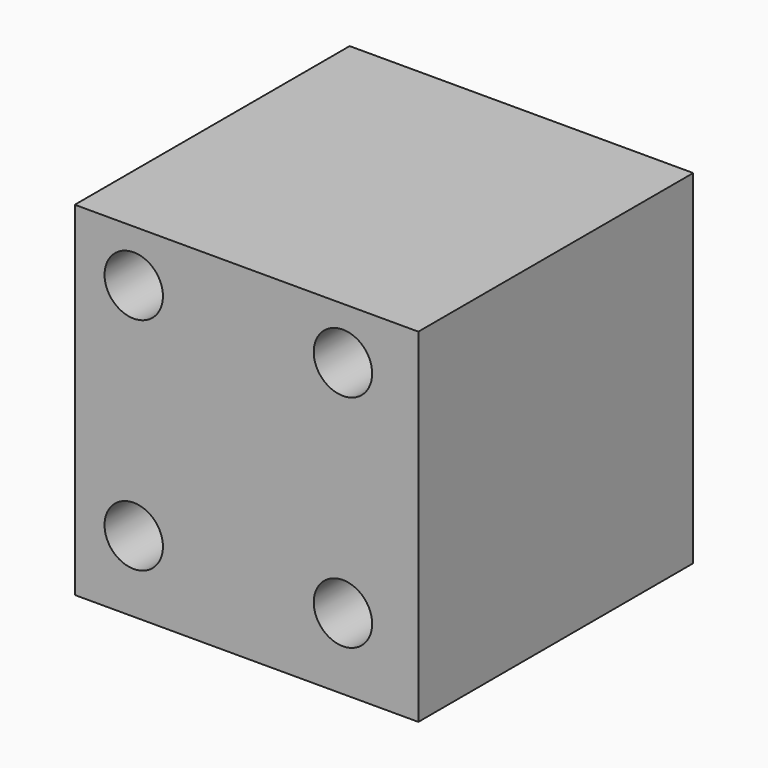
from build123d import *

# Parameters (mm, degrees)
F0_W     = 100
F0_H     = 100
F1_DEPTH = 100
F2_R     = 8.5
F3_DEPTH = 64
F5_ANGLE = 180


# Not quite as in the source:
# - a feature names something its author has since deleted; it is built from what else it names


with BuildPart() as f1:
    # F0 (on Front) → F1 (new body)
    with BuildSketch(Plane.XZ):
        with Locations((2.3967929184, 13.6052064598)):
            Rectangle(F0_W, F0_H)
    extrude(amount=F1_DEPTH)

    # F2 (on face) → F3 (cut)
    with BuildSketch(Plane.XZ.offset(100)):
        with Locations((30.443597585, 48.4984777868)):
            Circle(F2_R)
        with Locations((-30.443597585, -15.6539641321)):
            Circle(F2_R)
        with Locations((30.443597585, -15.6539641321)):
            Circle(F2_R)
        with Locations((-30.443597585, 48.4984777868)):
            Circle(F2_R)
    extrude(amount=-F3_DEPTH, mode=Mode.SUBTRACT)

    # F4 (on face) → F5 (revolve, cut)
    with BuildSketch(Plane.XZ.offset(100)):
        with BuildLine():
            Line((0, 0), (0, 26.83))
            ThreePointArc((0, 26.83), (-13.415, 13.415), (0, 0))
        make_face()
    revolve(axis=Axis((0, -100, 14.3139522988), (0, 0, 1)), revolution_arc=F5_ANGLE, mode=Mode.SUBTRACT)


solid = f1.part
